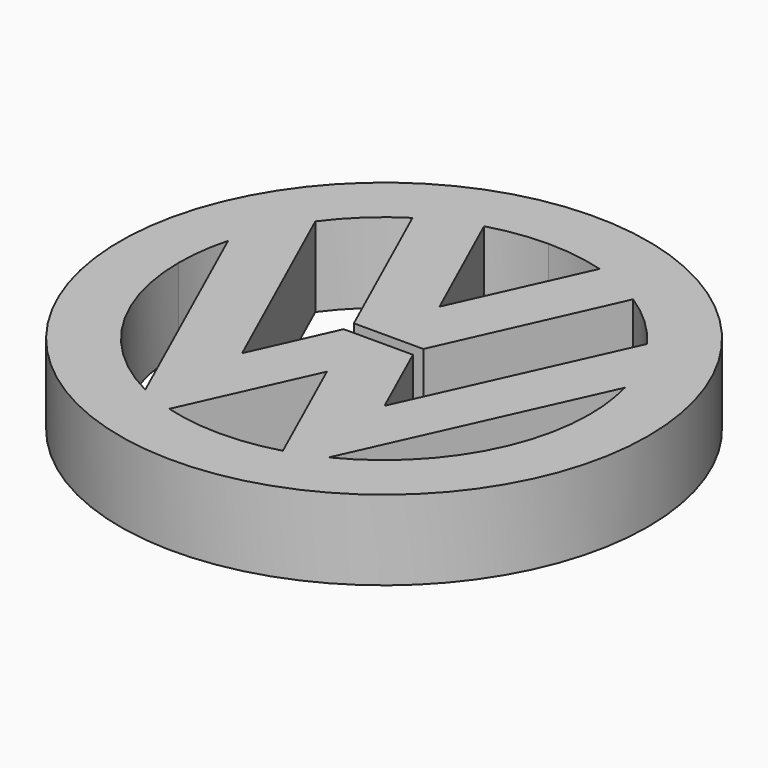
from build123d import *

# Parameters (mm, degrees)
F1_DEPTH = 25


# Not quite as in the source:
# - ends of sketch curves that miss each other by under 0.0002 mm in the source are joined


with BuildPart() as f1:
    # F0 (on Top) → F1 (new body)
    with BuildSketch(Plane.XY):
        with BuildLine():
            ThreePointArc((-82.6844, 0), (0, -82.6844), (82.6844, 0))
            ThreePointArc((82.6844, 0), (0, 82.6844), (-82.6844, 0))
        make_face()
        with BuildLine():
            ThreePointArc((-0.0001019994, -64.3575904446), (-8.9899783863, -63.7364917021), (-17.8043990333, -61.8630911161))
            Line((-17.8043990333, -61.8630911161), (0, -22.3774))
            Line((0, -22.3774), (17.7835, -61.8695))
            ThreePointArc((17.7835, -61.8695), (8.9783061535, -63.7325605397), (-0.0001019994, -64.3575904446))
        make_face(mode=Mode.SUBTRACT)
        with BuildLine():
            ThreePointArc((-64.3576040742, 5e-06), (-63.8166972636, 8.3999218175), (-62.181104878, 16.6567989674))
            Line((-62.181104878, 16.6567989674), (-28.7278, -57.6069))
            ThreePointArc((-28.7278, -57.6069), (-54.7289693105, -33.866650173), (-64.3576040742, 5e-06))
        make_face(mode=Mode.SUBTRACT)
        with BuildLine():
            ThreePointArc((64.356106725, 9e-06), (54.7239343065, -33.864451622), (28.7263060265, -57.6068980531))
            Line((28.7263060265, -57.6068980531), (62.2183, 16.5153))
            ThreePointArc((62.2183, 16.5153), (63.8186125658, 8.3264340159), (64.356106725, 9e-06))
        make_face(mode=Mode.SUBTRACT)
        with BuildLine():
            Line((0, 21.6991), (-18.1035, 61.7762))
            ThreePointArc((-18.1035, 61.7762), (-9.143995, 63.7130624999), (-9.9e-05, 64.355997063))
            ThreePointArc((-9.9e-05, 64.355997063), (9.132463164, 63.7090225476), (18.0825989725, 61.7810009054))
            Line((18.0825989725, 61.7810009054), (0, 21.6991))
        make_face(mode=Mode.SUBTRACT)
        with BuildLine():
            Line((10.9234, 1.7325), (34.545, 54.3084))
            ThreePointArc((34.545, 54.3084), (44.0251133087, 46.9417504609), (51.9809939632, 37.9504079731))
            Line((51.9809939632, 37.9504079731), (22.3019, -27.7266))
            Line((22.3019, -27.7266), (10.8496, -2.2616))
            Line((10.8496, -2.2616), (-10.8494, -2.2616))
            Line((-10.8494, -2.2616), (-22.3016, -27.7266))
            Line((-22.3016, -27.7266), (-51.9378, 38.0118))
            ThreePointArc((-51.9378, 38.0118), (-44.0003546147, 46.9677472651), (-34.5479019666, 54.3069079476))
            Line((-34.5479019666, 54.3069079476), (-10.8494, 1.7325))
            Line((-10.8494, 1.7325), (10.9234, 1.7325))
        make_face(mode=Mode.SUBTRACT)
    extrude(amount=F1_DEPTH)


solid = f1.part
